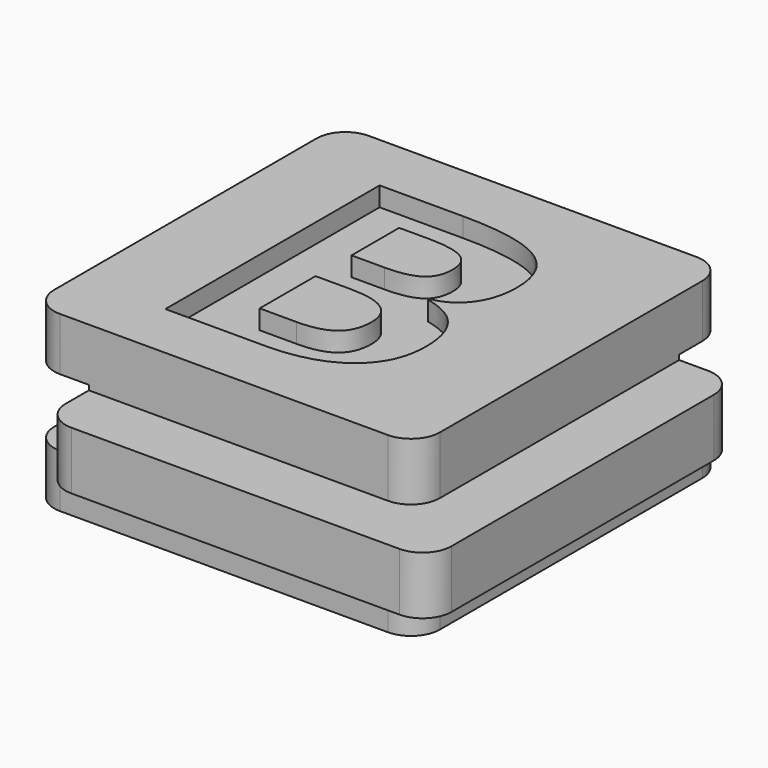
from build123d import *

# Parameters (mm, degrees)
F0_W         = 14
F0_H         = 3
F0_W_2       = 3
F1_DEPTH     = 20
F2_DEPTH     = 3
F3_W         = 3
F3_H         = 3
F4_DEPTH     = 100
F5_W         = 3
F5_H         = 3.5
F6_DEPTH     = 100
F7_R         = 1.5
F8_TEXT_SIZE = 19.4444444444
F9_DEPTH     = 1


# Not quite as in the source:
# - Text() gives the source's letters only with a copy of the font that has no kerning and outlines rounded to 1/6400 em; it was checked with that copy


with BuildPart() as f1:
    # F0 (on Front) → F1 (new body)
    with BuildSketch(Plane.XZ):
        Polygon((10, 1.5), (10, 4.5), (-10, 4.5), (-10, 1.5), (-7, 1.5), (7, 1.5), align=None)
        Rectangle(F0_W, F0_H)
        with Locations((11.5, 0)):
            Rectangle(F0_W_2, F0_H)
        with Locations((8.5, 0)):
            Rectangle(F0_W_2, F0_H)
        with Locations((-8.5, 0)):
            Rectangle(F0_W_2, F0_H)
        Polygon((10, -4.5), (10, -1.5), (7, -1.5), (-7, -1.5), (-10, -1.5), (-10, -4.5), align=None)
    extrude(amount=-F1_DEPTH)

    # F0 (on Front) → F2 (join)
    with BuildSketch(Plane.XZ):
        with Locations((-8.5, 0)):
            Rectangle(F0_W_2, F0_H)
        Rectangle(F0_W, F0_H)
        with Locations((8.5, 0)):
            Rectangle(F0_W_2, F0_H)
        with Locations((11.5, 0)):
            Rectangle(F0_W_2, F0_H)
    extrude(amount=F2_DEPTH)

    # F3 (on face) → F4 (cut)
    with BuildSketch(Plane.YZ.offset(13)):
        Polygon((23, -1.75), (23, 1.75), (17, 1.75), (17, 1.5), (20, 1.5), (20, -1.5), (17, -1.5), (17, -1.75), align=None)
        with Locations((18.5, 0)):
            Rectangle(F3_W, F3_H)
    extrude(amount=-F4_DEPTH, mode=Mode.SUBTRACT)

    # F5 (on face) → F6 (cut)
    with BuildSketch(Plane(origin=(0, 17, 0), x_dir=(-1, 0, 0), z_dir=(0, 1, 0))):
        with Locations((11.5, 0)):
            Rectangle(F5_W, F5_H)
        with Locations((8.5, 0)):
            Rectangle(F5_W, F5_H)
    extrude(amount=-F6_DEPTH, mode=Mode.SUBTRACT)

    # F7
    f7_edges = [f1.edges().sort_by_distance(p)[0] for p in [
        (-7, -3, 0),
        (13, -3, 0),
        (10, 0, 3),
        (10, 0, -3),
        (-10, 0, -3.125),
        (-10, 0, 3.125),
        (-7, 17, 0),
        (-10, 20, 3.125),
        (-10, 20, -3.125),
        (13, 17, 0),
        (10, 20, 3.125),
        (10, 20, -3.125),
    ]]
    fillet(f7_edges, radius=F7_R)

    # F8 (on face) → F9 (cut)
    with BuildSketch(Plane.XY.offset(4.5)):
        with Locations((-7.1801951318, 3)):
            Text('B', F8_TEXT_SIZE, font='Open Sans', font_style=FontStyle.BOLD, text_align=(TextAlign.LEFT, TextAlign.BOTTOM))
    extrude(amount=-F9_DEPTH, mode=Mode.SUBTRACT)


solid = f1.part
